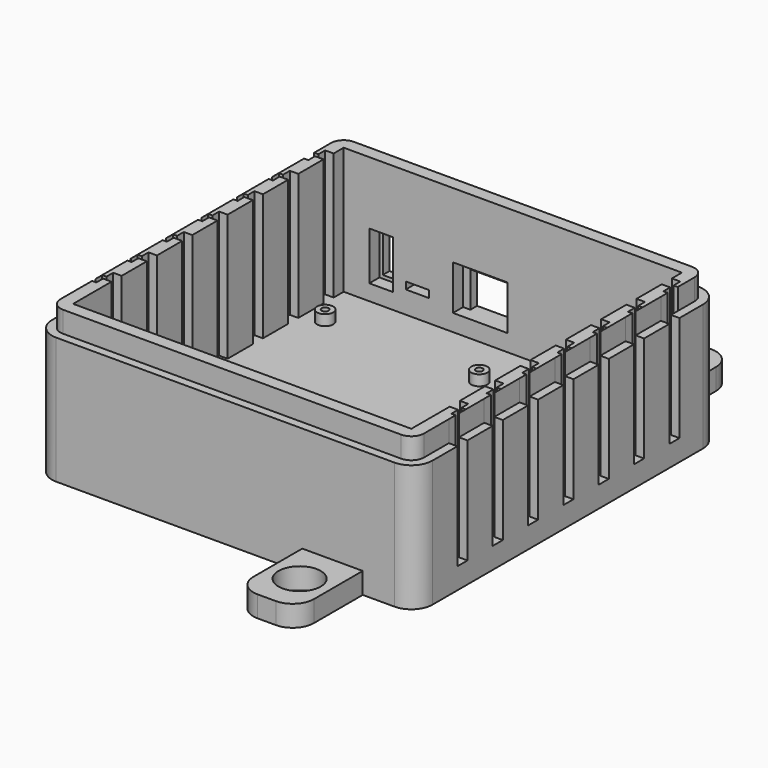
from build123d import *

# Parameters (mm, degrees)
F0_W      = 18.1644260883
F0_H      = 3.81
F0_H_2    = 2.54
F0_R      = 6.35
F0_W_2    = 2.5400000004
F0_H_3    = 9.4579567563
F0_W_3    = 2.54
F1_DEPTH  = 6.35
F2_DEPTH  = 38.1
F3_DEPTH  = 31.75
F0_R_2    = 2.4214450797
F0_R_3    = 1.0414
F4_DEPTH  = 6.35
F5_DEPTH  = 3.175
F6_W      = 7.0993
F6_H      = 14.50086
F6_W_2    = 5.1308
F6_H_2    = 12.5222
F7_DEPTH  = 3.81
F6_W_3    = 10.16
F6_H_3    = 6.096
F6_W_4    = 6.9088
F6_H_4    = 2.13106
F6_W_5    = 12.0142
F6_H_5    = 10.6934
F8_DEPTH  = 6.35
F9_DEPTH  = 3.81
F10_DEPTH = 38.1


# Not quite as in the source:
# - a feature names something its author has since deleted; it is built from what else it names


with BuildPart() as f1:
    # F0 (on Top) → F1 (new body)
    with BuildSketch(Plane.XY):
        with BuildLine():
            Line((23.1174400568, 54.61), (23.1174400568, 57.15))
            Line((23.1174400568, 57.15), (-50.8, 57.15))
            ThreePointArc((-50.8, 57.15), (-55.2901280605, 55.2901280605), (-57.15, 50.8))
            Line((-57.15, 50.8), (-57.15, 41.9416120576))
            Line((-57.15, 41.9416120576), (-54.61, 41.9416120576))
            Line((-54.61, 41.9416120576), (-54.61, 44.4816122126))
            Line((-54.61, 44.4816122126), (-54.61, 50.8))
            ThreePointArc((-54.61, 50.8), (-53.4940768363, 53.4940768363), (-50.8, 54.61))
            Line((-50.8, 54.61), (23.1174400568, 54.61))
        make_face()
        with BuildLine():
            Line((23.1174400568, 50.8), (23.1174400568, 54.61))
            Line((23.1174400568, 54.61), (-50.8, 54.61))
            ThreePointArc((-50.8, 54.61), (-53.4940768363, 53.4940768363), (-54.61, 50.8))
            Line((-54.61, 50.8), (-54.61, 44.4816122126))
            Line((-54.61, 44.4816122126), (-53.3399999996, 44.4816122126))
            Line((-53.3399999996, 44.4816122126), (-53.3399999996, 47.0216122126))
            Line((-53.3399999996, 47.0216122126), (-50.8, 47.0216122126))
            Line((-50.8, 47.0216122126), (-50.8, 50.8))
            Line((-50.8, 50.8), (23.1174400568, 50.8))
        make_face()
        with Locations((32.199653101, 52.705)):
            Rectangle(F0_W, F0_H)
        with Locations((32.199653101, 55.88)):
            Rectangle(F0_W, F0_H_2)
        with BuildLine():
            Line((23.1174400568, 57.15), (41.2818661451, 57.15))
            Line((41.2818661451, 57.15), (41.2818661451, 75.5032065153))
            ThreePointArc((41.2818661451, 75.5032065153), (39.4219942057, 79.9933345758), (34.9318661451, 81.8532065153))
            Line((34.9318661451, 81.8532065153), (29.4674400568, 81.8532065153))
            ThreePointArc((29.4674400568, 81.8532065153), (24.9773119963, 79.9933345758), (23.1174400568, 75.5032065153))
            Line((23.1174400568, 75.5032065153), (23.1174400568, 57.15))
        make_face()
        with Locations((32.199653101, 69.5016032577)):
            Circle(F0_R, mode=Mode.SUBTRACT)
        with BuildLine():
            ThreePointArc((57.15, 50.8), (55.2901280605, 55.2901280605), (50.8, 57.15))
            Line((50.8, 57.15), (41.2818661451, 57.15))
            Line((41.2818661451, 57.15), (41.2818661451, 54.61))
            Line((41.2818661451, 54.61), (50.8, 54.61))
            ThreePointArc((50.8, 54.61), (53.4940768363, 53.4940768363), (54.61, 50.8))
            Line((54.61, 50.8), (54.61, 44.4816122126))
            Line((54.61, 44.4816122126), (54.61, 41.9416120576))
            Line((54.61, 41.9416120576), (57.15, 41.9416120576))
            Line((57.15, 41.9416120576), (57.15, 50.8))
        make_face()
        with BuildLine():
            Line((50.8, 54.61), (41.2818661451, 54.61))
            Line((41.2818661451, 54.61), (41.2818661451, 50.8))
            Line((41.2818661451, 50.8), (50.8, 50.8))
            Line((50.8, 50.8), (50.8, 47.0216122126))
            Line((50.8, 47.0216122126), (53.3399999996, 47.0216122126))
            Line((53.3399999996, 47.0216122126), (53.3399999996, 44.4816122126))
            Line((53.3399999996, 44.4816122126), (54.61, 44.4816122126))
            Line((54.61, 44.4816122126), (54.61, 50.8))
            ThreePointArc((54.61, 50.8), (53.4940768363, 53.4940768363), (50.8, 54.61))
        make_face()
        Polygon((54.61, 40.6716121353), (54.61, 41.9416120576), (54.61, 44.4816122126), (53.3399999996, 44.4816122126), (53.3399999996, 47.0216122126), (50.8, 47.0216122126), (50.8, 43.2116121353), (53.3399999996, 43.2116121353), (53.3399999996, 40.6716121353), align=None)
        Polygon((57.15, 38.1316120576), (57.15, 41.9416120576), (54.61, 41.9416120576), (54.61, 40.6716121353), (54.6099999996, 38.1316120576), align=None)
        with Locations((55.8799999998, 33.4026336794)):
            Rectangle(F0_W_2, F0_H_3)
        Polygon((54.61, 28.6736553012), (54.61, 38.1316120576), (54.6099999996, 40.6716121353), (53.3399999996, 40.6716121353), (53.3399999996, 43.2116121353), (50.8, 43.2116121353), (50.8, 33.7536554562), (53.338121421, 33.7536554562), (53.338121421, 31.2136554562), (54.6081214215, 31.2136554562), (54.6081214215, 28.6736553012), align=None)
        Polygon((54.61, 24.8636553012), (54.61, 28.6736553012), (54.6081214215, 28.6736553012), (54.6081214215, 31.2136554562), (53.338121421, 31.2136554562), (53.338121421, 33.7536554562), (50.8, 33.7536554562), (50.8, 29.943655379), (53.338121421, 29.943655379), (53.338121421, 27.403655379), (54.608121421, 27.403655379), (54.608121421, 24.8636553012), align=None)
        with Locations((55.88, 26.7686553012)):
            Rectangle(F0_W_3, F0_H)
        with Locations((55.88, 20.1346769231)):
            Rectangle(F0_W_3, F0_H_3)
        Polygon((54.61, 15.4056985449), (54.61, 24.8636553012), (54.608121421, 24.8636553012), (54.608121421, 27.403655379), (53.338121421, 27.403655379), (53.338121421, 29.943655379), (50.8, 29.943655379), (50.8, 20.4856986999), (53.3362428425, 20.4856986999), (53.3362428425, 17.9456986999), (54.6062428429, 17.9456986999), (54.6062428429, 15.4056985449), align=None)
        Polygon((54.61, 11.5956985449), (54.61, 15.4056985449), (54.6062428429, 15.4056985449), (54.6062428429, 17.9456986999), (53.3362428425, 17.9456986999), (53.3362428425, 20.4856986999), (50.8, 20.4856986999), (50.8, 16.6756986226), (53.3362428425, 16.6756986226), (53.3362428425, 14.1356986226), (54.6062428424, 14.1356986226), (54.6062428424, 11.5956985449), align=None)
        with Locations((55.88, 13.5006985449)):
            Rectangle(F0_W_3, F0_H)
        Polygon((54.61, 2.1377417885), (54.61, 11.5956985449), (54.6062428424, 11.5956985449), (54.6062428424, 14.1356986226), (53.3362428425, 14.1356986226), (53.3362428425, 16.6756986226), (50.8, 16.6756986226), (50.8, 7.2177419435), (53.3343642639, 7.2177419435), (53.3343642639, 4.6777419435), (54.6043642643, 4.6777419435), (54.6043642643, 2.1377417885), align=None)
        with Locations((55.88, 6.8667201667)):
            Rectangle(F0_W_3, F0_H_3)
        with Locations((55.88, 0.2327417885)):
            Rectangle(F0_W_3, F0_H)
        Polygon((54.61, -1.6722582115), (54.61, 2.1377417885), (54.6043642643, 2.1377417885), (54.6043642643, 4.6777419435), (53.3343642639, 4.6777419435), (53.3343642639, 7.2177419435), (50.8, 7.2177419435), (50.8, 3.4077418663), (53.3343642639, 3.4077418663), (53.3343642639, 0.8677418663), (54.6043642639, 0.8677418663), (54.6043642639, -1.6722582115), align=None)
        Polygon((54.61, -11.1302149678), (54.61, -1.6722582115), (54.6043642639, -1.6722582115), (54.6043642639, 0.8677418663), (53.3343642639, 0.8677418663), (53.3343642639, 3.4077418663), (50.8, 3.4077418663), (50.8, -6.0502148128), (53.3324856854, -6.0502148128), (53.3324856854, -8.5902148128), (54.6024856858, -8.5902148128), (54.6024856858, -11.1302149678), align=None)
        with Locations((55.88, -6.4012365896)):
            Rectangle(F0_W_3, F0_H_3)
        Polygon((54.61, -14.9402149678), (54.61, -11.1302149678), (54.6024856858, -11.1302149678), (54.6024856858, -8.5902148128), (53.3324856854, -8.5902148128), (53.3324856854, -6.0502148128), (50.8, -6.0502148128), (50.8, -9.8602148901), (53.3324856853, -9.8602148901), (53.3324856853, -12.4002148901), (54.6024856853, -12.4002148901), (54.6024856853, -14.9402149678), align=None)
        with Locations((55.88, -13.0352149678)):
            Rectangle(F0_W_3, F0_H)
        with Locations((55.88, -19.669193346)):
            Rectangle(F0_W_3, F0_H_3)
        Polygon((54.61, -24.3981717241), (54.61, -14.9402149678), (54.6024856853, -14.9402149678), (54.6024856853, -12.4002148901), (53.3324856853, -12.4002148901), (53.3324856853, -9.8602148901), (50.8, -9.8602148901), (50.8, -19.3181715692), (53.3306071068, -19.3181715692), (53.3306071068, -21.8581715692), (54.6006071072, -21.8581715692), (54.6006071072, -24.3981717241), align=None)
        Polygon((54.61, -28.2081717241), (54.61, -24.3981717241), (54.6006071072, -24.3981717241), (54.6006071072, -21.8581715692), (53.3306071068, -21.8581715692), (53.3306071068, -19.3181715692), (50.8, -19.3181715692), (50.8, -23.1281716464), (53.3306071068, -23.1281716464), (53.3306071068, -25.6681716464), (54.6006071068, -25.6681716464), (54.6006071068, -28.2081717241), align=None)
        with Locations((55.88, -26.3031717241)):
            Rectangle(F0_W_3, F0_H)
        with Locations((55.88, -32.9371501023)):
            Rectangle(F0_W_3, F0_H_3)
        Polygon((54.61, -37.6661284805), (54.61, -28.2081717241), (54.6006071068, -28.2081717241), (54.6006071068, -25.6681716464), (53.3306071068, -25.6681716464), (53.3306071068, -23.1281716464), (50.8, -23.1281716464), (50.8, -32.5861283255), (53.3287285283, -32.5861283255), (53.3287285283, -35.1261283255), (54.5987285287, -35.1261283255), (54.5987285287, -37.6661284805), align=None)
        Polygon((54.61, -41.4761284805), (54.61, -37.6661284805), (54.5987285287, -37.6661284805), (54.5987285287, -35.1261283255), (53.3287285283, -35.1261283255), (53.3287285283, -32.5861283255), (50.8, -32.5861283255), (50.8, -36.3961284028), (53.3287285282, -36.3961284028), (53.3287285282, -38.9361284028), (54.5987285282, -38.9361284028), (54.5987285282, -41.4761284805), align=None)
        with Locations((55.88, -39.5711284805)):
            Rectangle(F0_W_3, F0_H)
        with BuildLine():
            Line((57.15, -50.8), (57.15, -41.4761284805))
            Line((57.15, -41.4761284805), (54.61, -41.4761284805))
            Line((54.61, -41.4761284805), (54.61, -50.8))
            ThreePointArc((54.61, -50.8), (53.4940768363, -53.4940768363), (50.8, -54.61))
            Line((50.8, -54.61), (41.2818661451, -54.61))
            Line((41.2818661451, -54.61), (41.2818661451, -57.15))
            Line((41.2818661451, -57.15), (50.8, -57.15))
            ThreePointArc((50.8, -57.15), (55.2901280605, -55.2901280605), (57.15, -50.8))
        make_face()
        with Locations((32.199653101, -52.705)):
            Rectangle(F0_W, F0_H)
        with Locations((32.199653101, -55.88)):
            Rectangle(F0_W, F0_H_2)
        with BuildLine():
            Line((41.2818661451, -75.5032065153), (41.2818661451, -57.15))
            Line((41.2818661451, -57.15), (23.1174400568, -57.15))
            Line((23.1174400568, -57.15), (23.1174400568, -75.5032065153))
            ThreePointArc((23.1174400568, -75.5032065153), (24.9773119963, -79.9933345758), (29.4674400568, -81.8532065153))
            Line((29.4674400568, -81.8532065153), (34.9318661451, -81.8532065153))
            ThreePointArc((34.9318661451, -81.8532065153), (39.4219942057, -79.9933345758), (41.2818661451, -75.5032065153))
        make_face()
        with Locations((32.199653101, -69.5016032577)):
            Circle(F0_R, mode=Mode.SUBTRACT)
        with BuildLine():
            Line((-54.5987285282, -41.4761284805), (-54.61, -41.4761284805))
            Line((-54.61, -41.4761284805), (-54.61, -50.8))
            ThreePointArc((-54.61, -50.8), (-53.4940768363, -53.4940768363), (-50.8, -54.61))
            Line((-50.8, -54.61), (23.1174400568, -54.61))
            Line((23.1174400568, -54.61), (23.1174400568, -50.8))
            Line((23.1174400568, -50.8), (-50.8, -50.8))
            Line((-50.8, -50.8), (-50.8, -36.3961284028))
            Line((-50.8, -36.3961284028), (-53.3287285282, -36.3961284028))
            Line((-53.3287285282, -36.3961284028), (-53.3287285282, -38.9361284028))
            Line((-53.3287285282, -38.9361284028), (-54.5987285282, -38.9361284028))
            Line((-54.5987285282, -38.9361284028), (-54.5987285282, -41.4761284805))
        make_face()
        with BuildLine():
            Line((-54.61, -41.4761284805), (-57.15, -41.4761284805))
            Line((-57.15, -41.4761284805), (-57.15, -50.8))
            ThreePointArc((-57.15, -50.8), (-55.2901280605, -55.2901280605), (-50.8, -57.15))
            Line((-50.8, -57.15), (23.1174400568, -57.15))
            Line((23.1174400568, -57.15), (23.1174400568, -54.61))
            Line((23.1174400568, -54.61), (-50.8, -54.61))
            ThreePointArc((-50.8, -54.61), (-53.4940768363, -53.4940768363), (-54.61, -50.8))
            Line((-54.61, -50.8), (-54.61, -41.4761284805))
        make_face()
        with Locations((-55.88, -39.5711284805)):
            Rectangle(F0_W_3, F0_H)
        Polygon((-54.5987285287, -37.6661284805), (-54.61, -37.6661284805), (-54.61, -41.4761284805), (-54.5987285282, -41.4761284805), (-54.5987285282, -38.9361284028), (-53.3287285282, -38.9361284028), (-53.3287285282, -36.3961284028), (-50.8, -36.3961284028), (-50.8, -32.5861283255), (-53.3287285283, -32.5861283255), (-53.3287285283, -35.1261283255), (-54.5987285287, -35.1261283255), align=None)
        with Locations((-55.88, -32.9371501023)):
            Rectangle(F0_W_3, F0_H_3)
        Polygon((-54.6006071068, -28.2081717241), (-54.61, -28.2081717241), (-54.61, -37.6661284805), (-54.5987285287, -37.6661284805), (-54.5987285287, -35.1261283255), (-53.3287285283, -35.1261283255), (-53.3287285283, -32.5861283255), (-50.8, -32.5861283255), (-50.8, -23.1281716464), (-53.3306071068, -23.1281716464), (-53.3306071068, -25.6681716464), (-54.6006071068, -25.6681716464), align=None)
        with Locations((-55.88, -26.3031717241)):
            Rectangle(F0_W_3, F0_H)
        Polygon((-54.6006071072, -24.3981717241), (-54.61, -24.3981717241), (-54.61, -28.2081717241), (-54.6006071068, -28.2081717241), (-54.6006071068, -25.6681716464), (-53.3306071068, -25.6681716464), (-53.3306071068, -23.1281716464), (-50.8, -23.1281716464), (-50.8, -19.3181715692), (-53.3306071068, -19.3181715692), (-53.3306071068, -21.8581715692), (-54.6006071072, -21.8581715692), align=None)
        with Locations((-55.88, -19.669193346)):
            Rectangle(F0_W_3, F0_H_3)
        Polygon((-54.6024856853, -14.9402149678), (-54.61, -14.9402149678), (-54.61, -24.3981717241), (-54.6006071072, -24.3981717241), (-54.6006071072, -21.8581715692), (-53.3306071068, -21.8581715692), (-53.3306071068, -19.3181715692), (-50.8, -19.3181715692), (-50.8, -9.8602148901), (-53.3324856853, -9.8602148901), (-53.3324856853, -12.4002148901), (-54.6024856853, -12.4002148901), align=None)
        with Locations((-55.88, -13.0352149678)):
            Rectangle(F0_W_3, F0_H)
        Polygon((-54.6024856858, -11.1302149678), (-54.61, -11.1302149678), (-54.61, -14.9402149678), (-54.6024856853, -14.9402149678), (-54.6024856853, -12.4002148901), (-53.3324856853, -12.4002148901), (-53.3324856853, -9.8602148901), (-50.8, -9.8602148901), (-50.8, -6.0502148128), (-53.3324856854, -6.0502148128), (-53.3324856854, -8.5902148128), (-54.6024856858, -8.5902148128), align=None)
        Polygon((-54.6043642639, -1.6722582115), (-54.61, -1.6722582115), (-54.61, -11.1302149678), (-54.6024856858, -11.1302149678), (-54.6024856858, -8.5902148128), (-53.3324856854, -8.5902148128), (-53.3324856854, -6.0502148128), (-50.8, -6.0502148128), (-50.8, 3.4077418663), (-53.3343642639, 3.4077418663), (-53.3343642639, 0.8677418663), (-54.6043642639, 0.8677418663), align=None)
        with Locations((-55.88, -6.4012365896)):
            Rectangle(F0_W_3, F0_H_3)
        with Locations((-55.88, 0.2327417885)):
            Rectangle(F0_W_3, F0_H)
        Polygon((-54.6043642643, 2.1377417885), (-54.61, 2.1377417885), (-54.61, -1.6722582115), (-54.6043642639, -1.6722582115), (-54.6043642639, 0.8677418663), (-53.3343642639, 0.8677418663), (-53.3343642639, 3.4077418663), (-50.8, 3.4077418663), (-50.8, 7.2177419435), (-53.3343642639, 7.2177419435), (-53.3343642639, 4.6777419435), (-54.6043642643, 4.6777419435), align=None)
        Polygon((-54.6062428424, 11.5956985449), (-54.61, 11.5956985449), (-54.61, 2.1377417885), (-54.6043642643, 2.1377417885), (-54.6043642643, 4.6777419435), (-53.3343642639, 4.6777419435), (-53.3343642639, 7.2177419435), (-50.8, 7.2177419435), (-50.8, 16.6756986226), (-53.3362428425, 16.6756986226), (-53.3362428425, 14.1356986226), (-54.6062428424, 14.1356986226), align=None)
        with Locations((-55.88, 6.8667201667)):
            Rectangle(F0_W_3, F0_H_3)
        with Locations((-55.88, 13.5006985449)):
            Rectangle(F0_W_3, F0_H)
        Polygon((-54.6062428429, 15.4056985449), (-54.61, 15.4056985449), (-54.61, 11.5956985449), (-54.6062428424, 11.5956985449), (-54.6062428424, 14.1356986226), (-53.3362428425, 14.1356986226), (-53.3362428425, 16.6756986226), (-50.8, 16.6756986226), (-50.8, 20.4856986999), (-53.3362428425, 20.4856986999), (-53.3362428425, 17.9456986999), (-54.6062428429, 17.9456986999), align=None)
        Polygon((-54.608121421, 24.8636553012), (-54.61, 24.8636553012), (-54.61, 15.4056985449), (-54.6062428429, 15.4056985449), (-54.6062428429, 17.9456986999), (-53.3362428425, 17.9456986999), (-53.3362428425, 20.4856986999), (-50.8, 20.4856986999), (-50.8, 29.943655379), (-53.338121421, 29.943655379), (-53.338121421, 27.403655379), (-54.608121421, 27.403655379), align=None)
        with Locations((-55.88, 20.1346769231)):
            Rectangle(F0_W_3, F0_H_3)
        with Locations((-55.88, 26.7686553012)):
            Rectangle(F0_W_3, F0_H)
        Polygon((-54.6081214215, 28.6736553012), (-54.61, 28.6736553012), (-54.61, 24.8636553012), (-54.608121421, 24.8636553012), (-54.608121421, 27.403655379), (-53.338121421, 27.403655379), (-53.338121421, 29.943655379), (-50.8, 29.943655379), (-50.8, 33.7536554562), (-53.338121421, 33.7536554562), (-53.338121421, 31.2136554562), (-54.6081214215, 31.2136554562), align=None)
        Polygon((-54.6099999996, 40.6716121353), (-54.6099999996, 38.1316120576), (-54.61, 28.6736553012), (-54.6081214215, 28.6736553012), (-54.6081214215, 31.2136554562), (-53.338121421, 31.2136554562), (-53.338121421, 33.7536554562), (-50.8, 33.7536554562), (-50.8, 43.2116121353), (-53.3399999996, 43.2116121353), (-53.3399999996, 40.6716121353), align=None)
        with Locations((-55.8799999998, 33.4026336794)):
            Rectangle(F0_W_2, F0_H_3)
        Polygon((-54.61, 41.9416120576), (-57.15, 41.9416120576), (-57.15, 38.1316120576), (-54.6099999996, 38.1316120576), (-54.6099999996, 40.6716121353), align=None)
        Polygon((-54.61, 44.4816122126), (-54.61, 41.9416120576), (-54.61, 40.6716121353), (-53.3399999996, 40.6716121353), (-53.3399999996, 43.2116121353), (-50.8, 43.2116121353), (-50.8, 47.0216122126), (-53.3399999996, 47.0216122126), (-53.3399999996, 44.4816122126), align=None)
    extrude(amount=-F1_DEPTH)

    # F0 (on Top) → F2 (join)
    with BuildSketch(Plane.XY):
        Polygon((54.61, 28.6736553012), (54.61, 38.1316120576), (54.6099999996, 40.6716121353), (53.3399999996, 40.6716121353), (53.3399999996, 43.2116121353), (50.8, 43.2116121353), (50.8, 33.7536554562), (53.338121421, 33.7536554562), (53.338121421, 31.2136554562), (54.6081214215, 31.2136554562), (54.6081214215, 28.6736553012), align=None)
        Polygon((54.61, 15.4056985449), (54.61, 24.8636553012), (54.608121421, 24.8636553012), (54.608121421, 27.403655379), (53.338121421, 27.403655379), (53.338121421, 29.943655379), (50.8, 29.943655379), (50.8, 20.4856986999), (53.3362428425, 20.4856986999), (53.3362428425, 17.9456986999), (54.6062428429, 17.9456986999), (54.6062428429, 15.4056985449), align=None)
        with Locations((32.199653101, 52.705)):
            Rectangle(F0_W, F0_H)
        Polygon((54.61, 2.1377417885), (54.61, 11.5956985449), (54.6062428424, 11.5956985449), (54.6062428424, 14.1356986226), (53.3362428425, 14.1356986226), (53.3362428425, 16.6756986226), (50.8, 16.6756986226), (50.8, 7.2177419435), (53.3343642639, 7.2177419435), (53.3343642639, 4.6777419435), (54.6043642643, 4.6777419435), (54.6043642643, 2.1377417885), align=None)
        Polygon((54.61, -11.1302149678), (54.61, -1.6722582115), (54.6043642639, -1.6722582115), (54.6043642639, 0.8677418663), (53.3343642639, 0.8677418663), (53.3343642639, 3.4077418663), (50.8, 3.4077418663), (50.8, -6.0502148128), (53.3324856854, -6.0502148128), (53.3324856854, -8.5902148128), (54.6024856858, -8.5902148128), (54.6024856858, -11.1302149678), align=None)
        Polygon((54.61, -24.3981717241), (54.61, -14.9402149678), (54.6024856853, -14.9402149678), (54.6024856853, -12.4002148901), (53.3324856853, -12.4002148901), (53.3324856853, -9.8602148901), (50.8, -9.8602148901), (50.8, -19.3181715692), (53.3306071068, -19.3181715692), (53.3306071068, -21.8581715692), (54.6006071072, -21.8581715692), (54.6006071072, -24.3981717241), align=None)
        Polygon((54.61, -37.6661284805), (54.61, -28.2081717241), (54.6006071068, -28.2081717241), (54.6006071068, -25.6681716464), (53.3306071068, -25.6681716464), (53.3306071068, -23.1281716464), (50.8, -23.1281716464), (50.8, -32.5861283255), (53.3287285283, -32.5861283255), (53.3287285283, -35.1261283255), (54.5987285287, -35.1261283255), (54.5987285287, -37.6661284805), align=None)
        with Locations((32.199653101, -52.705)):
            Rectangle(F0_W, F0_H)
        with BuildLine():
            Line((-54.5987285282, -41.4761284805), (-54.61, -41.4761284805))
            Line((-54.61, -41.4761284805), (-54.61, -50.8))
            ThreePointArc((-54.61, -50.8), (-53.4940768363, -53.4940768363), (-50.8, -54.61))
            Line((-50.8, -54.61), (23.1174400568, -54.61))
            Line((23.1174400568, -54.61), (23.1174400568, -50.8))
            Line((23.1174400568, -50.8), (-50.8, -50.8))
            Line((-50.8, -50.8), (-50.8, -36.3961284028))
            Line((-50.8, -36.3961284028), (-53.3287285282, -36.3961284028))
            Line((-53.3287285282, -36.3961284028), (-53.3287285282, -38.9361284028))
            Line((-53.3287285282, -38.9361284028), (-54.5987285282, -38.9361284028))
            Line((-54.5987285282, -38.9361284028), (-54.5987285282, -41.4761284805))
        make_face()
        Polygon((-54.6006071068, -28.2081717241), (-54.61, -28.2081717241), (-54.61, -37.6661284805), (-54.5987285287, -37.6661284805), (-54.5987285287, -35.1261283255), (-53.3287285283, -35.1261283255), (-53.3287285283, -32.5861283255), (-50.8, -32.5861283255), (-50.8, -23.1281716464), (-53.3306071068, -23.1281716464), (-53.3306071068, -25.6681716464), (-54.6006071068, -25.6681716464), align=None)
        Polygon((-54.6024856853, -14.9402149678), (-54.61, -14.9402149678), (-54.61, -24.3981717241), (-54.6006071072, -24.3981717241), (-54.6006071072, -21.8581715692), (-53.3306071068, -21.8581715692), (-53.3306071068, -19.3181715692), (-50.8, -19.3181715692), (-50.8, -9.8602148901), (-53.3324856853, -9.8602148901), (-53.3324856853, -12.4002148901), (-54.6024856853, -12.4002148901), align=None)
        Polygon((-54.6043642639, -1.6722582115), (-54.61, -1.6722582115), (-54.61, -11.1302149678), (-54.6024856858, -11.1302149678), (-54.6024856858, -8.5902148128), (-53.3324856854, -8.5902148128), (-53.3324856854, -6.0502148128), (-50.8, -6.0502148128), (-50.8, 3.4077418663), (-53.3343642639, 3.4077418663), (-53.3343642639, 0.8677418663), (-54.6043642639, 0.8677418663), align=None)
        Polygon((-54.6062428424, 11.5956985449), (-54.61, 11.5956985449), (-54.61, 2.1377417885), (-54.6043642643, 2.1377417885), (-54.6043642643, 4.6777419435), (-53.3343642639, 4.6777419435), (-53.3343642639, 7.2177419435), (-50.8, 7.2177419435), (-50.8, 16.6756986226), (-53.3362428425, 16.6756986226), (-53.3362428425, 14.1356986226), (-54.6062428424, 14.1356986226), align=None)
        Polygon((-54.608121421, 24.8636553012), (-54.61, 24.8636553012), (-54.61, 15.4056985449), (-54.6062428429, 15.4056985449), (-54.6062428429, 17.9456986999), (-53.3362428425, 17.9456986999), (-53.3362428425, 20.4856986999), (-50.8, 20.4856986999), (-50.8, 29.943655379), (-53.338121421, 29.943655379), (-53.338121421, 27.403655379), (-54.608121421, 27.403655379), align=None)
        Polygon((-54.6099999996, 40.6716121353), (-54.6099999996, 38.1316120576), (-54.61, 28.6736553012), (-54.6081214215, 28.6736553012), (-54.6081214215, 31.2136554562), (-53.338121421, 31.2136554562), (-53.338121421, 33.7536554562), (-50.8, 33.7536554562), (-50.8, 43.2116121353), (-53.3399999996, 43.2116121353), (-53.3399999996, 40.6716121353), align=None)
        with BuildLine():
            Line((23.1174400568, 50.8), (23.1174400568, 54.61))
            Line((23.1174400568, 54.61), (-50.8, 54.61))
            ThreePointArc((-50.8, 54.61), (-53.4940768363, 53.4940768363), (-54.61, 50.8))
            Line((-54.61, 50.8), (-54.61, 44.4816122126))
            Line((-54.61, 44.4816122126), (-53.3399999996, 44.4816122126))
            Line((-53.3399999996, 44.4816122126), (-53.3399999996, 47.0216122126))
            Line((-53.3399999996, 47.0216122126), (-50.8, 47.0216122126))
            Line((-50.8, 47.0216122126), (-50.8, 50.8))
            Line((-50.8, 50.8), (23.1174400568, 50.8))
        make_face()
        with BuildLine():
            Line((50.8, 54.61), (41.2818661451, 54.61))
            Line((41.2818661451, 54.61), (41.2818661451, 50.8))
            Line((41.2818661451, 50.8), (50.8, 50.8))
            Line((50.8, 50.8), (50.8, 47.0216122126))
            Line((50.8, 47.0216122126), (53.3399999996, 47.0216122126))
            Line((53.3399999996, 47.0216122126), (53.3399999996, 44.4816122126))
            Line((53.3399999996, 44.4816122126), (54.61, 44.4816122126))
            Line((54.61, 44.4816122126), (54.61, 50.8))
            ThreePointArc((54.61, 50.8), (53.4940768363, 53.4940768363), (50.8, 54.61))
        make_face()
    extrude(amount=F2_DEPTH)

    # F0 (on Top) → F3 (join)
    with BuildSketch(Plane.XY):
        with Locations((-55.8799999998, 33.4026336794)):
            Rectangle(F0_W_2, F0_H_3)
        with Locations((-55.88, 20.1346769231)):
            Rectangle(F0_W_3, F0_H_3)
        with Locations((-55.88, 6.8667201667)):
            Rectangle(F0_W_3, F0_H_3)
        with Locations((-55.88, -6.4012365896)):
            Rectangle(F0_W_3, F0_H_3)
        with Locations((-55.88, -19.669193346)):
            Rectangle(F0_W_3, F0_H_3)
        with Locations((-55.88, -32.9371501023)):
            Rectangle(F0_W_3, F0_H_3)
        with BuildLine():
            Line((23.1174400568, 54.61), (23.1174400568, 57.15))
            Line((23.1174400568, 57.15), (-50.8, 57.15))
            ThreePointArc((-50.8, 57.15), (-55.2901280605, 55.2901280605), (-57.15, 50.8))
            Line((-57.15, 50.8), (-57.15, 41.9416120576))
            Line((-57.15, 41.9416120576), (-54.61, 41.9416120576))
            Line((-54.61, 41.9416120576), (-54.61, 44.4816122126))
            Line((-54.61, 44.4816122126), (-54.61, 50.8))
            ThreePointArc((-54.61, 50.8), (-53.4940768363, 53.4940768363), (-50.8, 54.61))
            Line((-50.8, 54.61), (23.1174400568, 54.61))
        make_face()
        with BuildLine():
            Line((-54.61, -41.4761284805), (-57.15, -41.4761284805))
            Line((-57.15, -41.4761284805), (-57.15, -50.8))
            ThreePointArc((-57.15, -50.8), (-55.2901280605, -55.2901280605), (-50.8, -57.15))
            Line((-50.8, -57.15), (23.1174400568, -57.15))
            Line((23.1174400568, -57.15), (23.1174400568, -54.61))
            Line((23.1174400568, -54.61), (-50.8, -54.61))
            ThreePointArc((-50.8, -54.61), (-53.4940768363, -53.4940768363), (-54.61, -50.8))
            Line((-54.61, -50.8), (-54.61, -41.4761284805))
        make_face()
        with Locations((32.199653101, -55.88)):
            Rectangle(F0_W, F0_H_2)
        with BuildLine():
            Line((57.15, -50.8), (57.15, -41.4761284805))
            Line((57.15, -41.4761284805), (54.61, -41.4761284805))
            Line((54.61, -41.4761284805), (54.61, -50.8))
            ThreePointArc((54.61, -50.8), (53.4940768363, -53.4940768363), (50.8, -54.61))
            Line((50.8, -54.61), (41.2818661451, -54.61))
            Line((41.2818661451, -54.61), (41.2818661451, -57.15))
            Line((41.2818661451, -57.15), (50.8, -57.15))
            ThreePointArc((50.8, -57.15), (55.2901280605, -55.2901280605), (57.15, -50.8))
        make_face()
        with Locations((55.8799999998, 33.4026336794)):
            Rectangle(F0_W_2, F0_H_3)
        with Locations((55.88, 20.1346769231)):
            Rectangle(F0_W_3, F0_H_3)
        with Locations((55.88, 6.8667201667)):
            Rectangle(F0_W_3, F0_H_3)
        with Locations((55.88, -6.4012365896)):
            Rectangle(F0_W_3, F0_H_3)
        with Locations((55.88, -19.669193346)):
            Rectangle(F0_W_3, F0_H_3)
        with Locations((55.88, -32.9371501023)):
            Rectangle(F0_W_3, F0_H_3)
        with BuildLine():
            ThreePointArc((57.15, 50.8), (55.2901280605, 55.2901280605), (50.8, 57.15))
            Line((50.8, 57.15), (41.2818661451, 57.15))
            Line((41.2818661451, 57.15), (41.2818661451, 54.61))
            Line((41.2818661451, 54.61), (50.8, 54.61))
            ThreePointArc((50.8, 54.61), (53.4940768363, 53.4940768363), (54.61, 50.8))
            Line((54.61, 50.8), (54.61, 44.4816122126))
            Line((54.61, 44.4816122126), (54.61, 41.9416120576))
            Line((54.61, 41.9416120576), (57.15, 41.9416120576))
            Line((57.15, 41.9416120576), (57.15, 50.8))
        make_face()
        with Locations((32.199653101, 55.88)):
            Rectangle(F0_W, F0_H_2)
    extrude(amount=F3_DEPTH)

    # F0 (on Top) + F3_face (on face) → F4 (join)
    with BuildSketch(Plane.XY):
        Polygon((50.8, 50.8), (41.2818661451, 50.8), (23.1174400568, 50.8), (-50.8, 50.8), (-50.8, 47.0216122126), (-50.8, 43.2116121353), (-50.8, 33.7536554562), (-50.8, 29.943655379), (-50.8, 20.4856986999), (-50.8, 16.6756986226), (-50.8, 7.2177419435), (-50.8, 3.4077418663), (-50.8, -6.0502148128), (-50.8, -9.8602148901), (-50.8, -19.3181715692), (-50.8, -23.1281716464), (-50.8, -32.5861283255), (-50.8, -36.3961284028), (-50.8, -50.8), (23.1174400568, -50.8), (41.2818661451, -50.8), (50.8, -50.8), (50.8, -36.3961284028), (50.8, -32.5861283255), (50.8, -23.1281716464), (50.8, -19.3181715692), (50.8, -9.8602148901), (50.8, -6.0502148128), (50.8, 3.4077418663), (50.8, 7.2177419435), (50.8, 16.6756986226), (50.8, 20.4856986999), (50.8, 29.943655379), (50.8, 33.7536554562), (50.8, 43.2116121353), (50.8, 47.0216122126), align=None)
        with Locations((-39.6748, -15.7734)):
            Circle(F0_R_2, mode=Mode.SUBTRACT)
        with Locations((-11.7348, -15.7734)):
            Circle(F0_R_2, mode=Mode.SUBTRACT)
        with Locations((-44.7675, 36.29914)):
            Circle(F0_R_2, mode=Mode.SUBTRACT)
        with Locations((2.5527, 35.0266)):
            Circle(F0_R_2, mode=Mode.SUBTRACT)
        with BuildLine():
            Line((54.61, -50.8), (54.61, -41.4761284805))
            Line((54.61, -41.4761284805), (54.5987285282, -41.4761284805))
            Line((54.5987285282, -41.4761284805), (54.5987285282, -38.9361284028))
            Line((54.5987285282, -38.9361284028), (53.3287285282, -38.9361284028))
            Line((53.3287285282, -38.9361284028), (53.3287285282, -36.3961284028))
            Line((53.3287285282, -36.3961284028), (50.8, -36.3961284028))
            Line((50.8, -36.3961284028), (50.8, -50.8))
            Line((50.8, -50.8), (41.2818661451, -50.8))
            Line((41.2818661451, -50.8), (41.2818661451, -54.61))
            Line((41.2818661451, -54.61), (50.8, -54.61))
            ThreePointArc((50.8, -54.61), (53.4940768363, -53.4940768363), (54.61, -50.8))
        make_face()
        with Locations((-44.7675, 36.29914)):
            Circle(F0_R_2)
        with Locations((-44.7675, 36.29914)):
            Circle(F0_R_3, mode=Mode.SUBTRACT)
        with Locations((2.5527, 35.0266)):
            Circle(F0_R_2)
        with Locations((2.5527, 35.0266)):
            Circle(F0_R_3, mode=Mode.SUBTRACT)
        with Locations((-11.7348, -15.7734)):
            Circle(F0_R_2)
        with Locations((-11.7348, -15.7734)):
            Circle(F0_R_3, mode=Mode.SUBTRACT)
        with Locations((-39.6748, -15.7734)):
            Circle(F0_R_2)
        with Locations((-39.6748, -15.7734)):
            Circle(F0_R_3, mode=Mode.SUBTRACT)
        with Locations((-44.7675, 36.29914)):
            Circle(F0_R_3)
        with Locations((2.5527, 35.0266)):
            Circle(F0_R_3)
        with Locations((-11.7348, -15.7734)):
            Circle(F0_R_3)
        with Locations((-39.6748, -15.7734)):
            Circle(F0_R_3)
    with BuildSketch(Plane(origin=(0, -54.3378605157, 31.75), x_dir=(1, 0, 0), z_dir=(0, 0, 1))):
        with BuildLine():
            ThreePointArc((-50.8, -0.2721394843), (-53.4940768363, 0.8437836794), (-54.61, 3.5378605157))
            Line((-54.61, 3.5378605157), (-54.61, 12.8617320352))
            Line((-54.61, 12.8617320352), (-57.15, 12.8617320352))
            Line((-57.15, 12.8617320352), (-57.15, 3.5378605157))
            ThreePointArc((-57.15, 3.5378605157), (-55.2901280605, -0.9522675448), (-50.8, -2.8121394843))
            Line((-50.8, -2.8121394843), (50.8, -2.8121394843))
            ThreePointArc((50.8, -2.8121394843), (55.2901280605, -0.9522675448), (57.15, 3.5378605157))
            Line((57.15, 3.5378605157), (57.15, 12.8617320352))
            Line((57.15, 12.8617320352), (54.61, 12.8617320352))
            Line((54.61, 12.8617320352), (54.61, 3.5378605157))
            ThreePointArc((54.61, 3.5378605157), (53.4940768363, 0.8437836794), (50.8, -0.2721394843))
            Line((50.8, -0.2721394843), (41.2818661451, -0.2721394843))
            Line((41.2818661451, -0.2721394843), (-50.8, -0.2721394843))
        make_face()
    extrude(amount=-F4_DEPTH)

    # F0 (on Top) → F5 (join)
    with BuildSketch(Plane.XY):
        with Locations((-44.7675, 36.29914)):
            Circle(F0_R_2)
        with Locations((-44.7675, 36.29914)):
            Circle(F0_R_3, mode=Mode.SUBTRACT)
        with Locations((2.5527, 35.0266)):
            Circle(F0_R_2)
        with Locations((2.5527, 35.0266)):
            Circle(F0_R_3, mode=Mode.SUBTRACT)
        with Locations((-11.7348, -15.7734)):
            Circle(F0_R_2)
        with Locations((-11.7348, -15.7734)):
            Circle(F0_R_3, mode=Mode.SUBTRACT)
        with Locations((-39.6748, -15.7734)):
            Circle(F0_R_2)
        with Locations((-39.6748, -15.7734)):
            Circle(F0_R_3, mode=Mode.SUBTRACT)
    extrude(amount=F5_DEPTH)

    # F6 (on face) → F7 (cut)
    with BuildSketch(Plane.XZ.offset(-50.8)):
        with Locations((-39.55415, 11.98499)):
            Rectangle(F6_W, F6_H)
        with Locations((-39.5478, 11.98626)):
            Rectangle(F6_W_2, F6_H_2, mode=Mode.SUBTRACT)
        Polygon((-1.5875, 18.46326), (-17.97558, 18.46326), (-17.97558, 5.06984), (-15.79118, 5.06984), (-15.79118, 15.76324), (-3.77698, 15.76324), (-3.77698, 5.06984), (-1.5875, 5.06984), align=None)
    extrude(amount=-F7_DEPTH, mode=Mode.SUBTRACT)

    # F6 (on face) → F8 (cut)
    with BuildSketch(Plane.XZ.offset(-50.8)):
        with Locations((-39.5478, 11.98626)):
            Rectangle(F6_W_2, F6_H_2)
        with Locations((-28.70454, 7.72287)):
            Rectangle(F6_W_3, F6_H_3)
        with Locations((-28.70454, 7.72287)):
            Rectangle(F6_W_4, F6_H_4, mode=Mode.SUBTRACT)
        with Locations((-9.78408, 10.41654)):
            Rectangle(F6_W_5, F6_H_5)
        with Locations((-28.70454, 7.72287)):
            Rectangle(F6_W_4, F6_H_4)
    extrude(amount=-F8_DEPTH, mode=Mode.SUBTRACT)

    # F6 (on face) → F9 (join)
    with BuildSketch(Plane.XZ.offset(-50.8)):
        with Locations((-28.70454, 7.72287)):
            Rectangle(F6_W_3, F6_H_3)
        with Locations((-28.70454, 7.72287)):
            Rectangle(F6_W_4, F6_H_4, mode=Mode.SUBTRACT)
    extrude(amount=-F9_DEPTH)

    # F0 (on Top) → F10 (join)
    with BuildSketch(Plane.XY):
        with BuildLine():
            Line((54.61, -50.8), (54.61, -41.4761284805))
            Line((54.61, -41.4761284805), (54.5987285282, -41.4761284805))
            Line((54.5987285282, -41.4761284805), (54.5987285282, -38.9361284028))
            Line((54.5987285282, -38.9361284028), (53.3287285282, -38.9361284028))
            Line((53.3287285282, -38.9361284028), (53.3287285282, -36.3961284028))
            Line((53.3287285282, -36.3961284028), (50.8, -36.3961284028))
            Line((50.8, -36.3961284028), (50.8, -50.8))
            Line((50.8, -50.8), (41.2818661451, -50.8))
            Line((41.2818661451, -50.8), (41.2818661451, -54.61))
            Line((41.2818661451, -54.61), (50.8, -54.61))
            ThreePointArc((50.8, -54.61), (53.4940768363, -53.4940768363), (54.61, -50.8))
        make_face()
    extrude(amount=F10_DEPTH)


solid = f1.part
